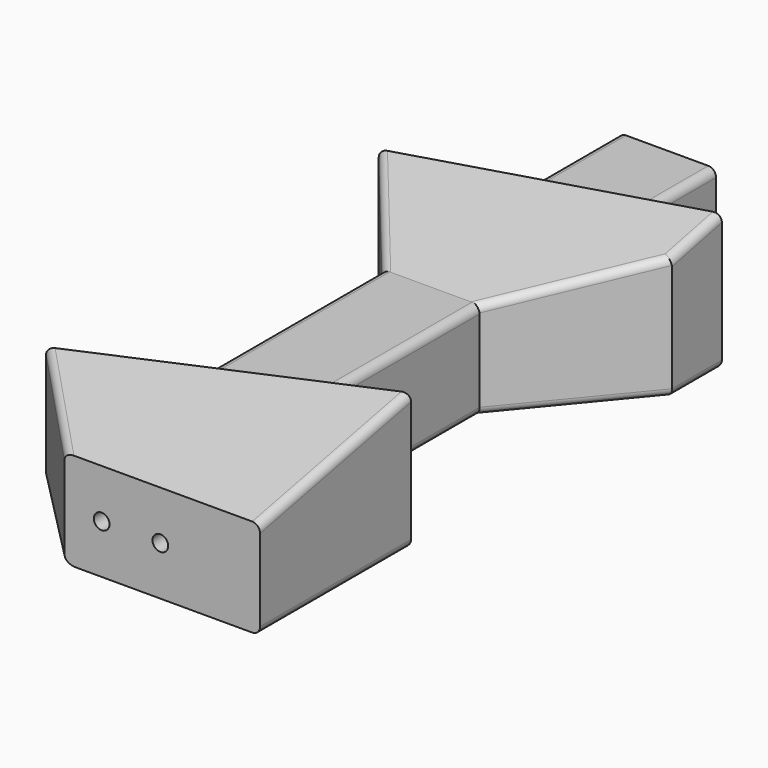
from build123d import *

# Parameters (mm, degrees)
F0_W           = 25
F0_H           = 33
F1_DEPTH       = 25
F3_DEPTH       = 10
F5_DEPTH       = 81.7
F7_DEPTH       = 10
F9_DEPTH       = 92
F10_W          = 13
F10_H          = 13
F11_DEPTH      = 135
F14_W          = 99.2073006928
F14_H          = 199.154949747
F15_DEPTH      = 88
F16_R          = 1.9
F17_DEPTH      = 7
F18_R          = 1.9
F19_DEPTH      = 7
F21_DEPTH      = 18
F22_T1_DEPTH   = 58.2865340729
F22_T3_DEPTH   = 59.3111485648
F22_T5_DEPTH   = 45.6084808239
F22_T7_DEPTH   = 44.6581070284
F22_T9_DEPTH   = 26.3114146799
F22_T11_DEPTH  = 25.9417421253
F22_T16_DEPTH  = 70.8165659944
F22_T23_DEPTH  = 70.8165659944
F22_T29_DEPTH  = 70.8165659944
F22_T35_DEPTH  = 78.4598330308
F22_T41_DEPTH  = 78.4598330308
F22_T47_DEPTH  = 78.4598330308
F22_T54_DEPTH  = 70.8165659944
F22_T60_DEPTH  = 78.4598330308
F22_T66_DEPTH  = 49.2253281189
F22_T71_DEPTH  = 48.4985768834
F22_T77_DEPTH  = 48.4985768834
F22_T83_DEPTH  = 48.4985768834
F22_T89_DEPTH  = 49.2253281189
F22_T94_DEPTH  = 48.4985768834
F22_T100_DEPTH = 48.4985768834
F22_T106_DEPTH = 48.4985768834
F22_T112_DEPTH = 44.6860859582
F22_T117_DEPTH = 50
F22_T122_DEPTH = 44.6860859582
F22_T127_DEPTH = 50
F22_T133_DEPTH = 70.8165659944
F22_T138_DEPTH = 48.4985768834
F22_T146_DEPTH = 48.4985768834
F22_T151_DEPTH = 78.4598330308
F22_T159_DEPTH = 70.8165659944
F22_T163_DEPTH = 49.2253281189
F22_T170_DEPTH = 49.2253281189
F22_T174_DEPTH = 78.4598330308


# Not quite as in the source:
# - a fillet or chamfer that OpenCascade refuses, or shapes differently, is made with other operations: its cross-section is extruded or revolved along the edge and cut away or added


with BuildPart() as f1:
    # F0 (on Top) → F1 (new body)
    with BuildSketch(Plane.XY):
        with Locations((12.5, 16.5)):
            Rectangle(F0_W, F0_H)
        Polygon((-25, 25.3567329635), (0, 0), (0, 33), align=None)
        with Locations((37.5, 16.5)):
            Rectangle(F0_W, F0_H)
        Polygon((25, 40.6432670365), (0, 33), (25, 33), align=None)
        Polygon((0, 101.4598330308), (0, 33), (25, 40.6432670365), (25, 101.4598330308), (25, 137), (0, 137), align=None)
        Polygon((25, 40.6432670365), (25, 33), (50, 33), (50, 48.2865340729), align=None)
        Polygon((-25, 131.6860859582), (0, 101.4598330308), (0, 137), align=None)
        Polygon((25, 137), (25, 101.4598330308), (50, 131.6860859582), (50, 147.6278280835), (25, 142.3139140418), align=None)
        Polygon((25, 142.3139140418), (0, 137), (25, 137), align=None)
        Polygon((0, 177), (0, 137), (25, 142.3139140418), (25, 177), align=None)
    extrude(amount=F1_DEPTH)

    # F2 (on face) → F3 (join)
    with BuildSketch(Plane(origin=(0, 0, 0), x_dir=(1, 0, 0), z_dir=(0, 0, -1))):
        Polygon((50, -131.6860859582), (25, -101.4598330308), (0, -101.4598330308), (-25, -131.6860859582), (50, -147.6278280835), align=None)
    extrude(amount=F3_DEPTH)

    # F4 (on face) → F5 (cut, symmetric)
    with BuildSketch(Plane.YZ.offset(25)):
        Polygon((101.4598330308, -21.1370438337), (147.6278330308, -10), (101.4598330308, 0), align=None)
    extrude(amount=F5_DEPTH, both=True, mode=Mode.SUBTRACT)

    # F6 (on face) → F7 (join)
    with BuildSketch(Plane(origin=(0, 0, 0), x_dir=(1, 0, 0), z_dir=(0, 0, -1))):
        Polygon((50, -48.2865340729), (50, 0), (0, 0), (-25, -25.3567329635), align=None)
    extrude(amount=F7_DEPTH)

    # F8 (on face) → F9 (cut)
    with BuildSketch(Plane.YZ.offset(50)):
        Polygon((48.2865340729, -10), (0, 0), (0, -39.534393698), (48.2865340729, -39.534393698), align=None)
    extrude(amount=-F9_DEPTH, mode=Mode.SUBTRACT)

    # F10 (on face) → F11 (cut)
    with BuildSketch(Plane(origin=(0, 177, 0), x_dir=(-1, 0, 0), z_dir=(0, 1, 0))):
        with Locations((-12.5, 12.5)):
            Rectangle(F10_W, F10_H)
    extrude(amount=-F11_DEPTH, mode=Mode.SUBTRACT)


with BuildPart() as f13_1:
    # F13: instance of F1
    add(f1.part.mirror(Plane(origin=(16.2715907381, 80.4050719696, 50), x_dir=(1, 0, 0), z_dir=(0, 0, 1))))

    # F16 (on face) → F17 (cut)
    with BuildSketch(Plane(origin=(-27.8614600507, 131.0778638485, 0), x_dir=(-0.9781476007, -0.2079116908, 0), z_dir=(-0.2079116908, 0.9781476007, 0))):
        with Locations((-18.6253867704, 87.5)):
            Circle(F16_R)
        with BuildLine():
            ThreePointArc((-72.2009313853, 87.5), (-70.3009313853, 85.6), (-68.4009313853, 87.5))
            ThreePointArc((-68.4009313853, 87.5), (-70.3009313853, 89.4), (-72.2009313853, 87.5))
        make_face()
    extrude(amount=-F17_DEPTH, mode=Mode.SUBTRACT)

    # F18 (on face) → F19 (cut)
    with BuildSketch(Plane(origin=(-9.2266829073, 30.1791199472, 0), x_dir=(-0.956304756, -0.2923717047, 0), z_dir=(-0.2923717047, 0.956304756, 0))):
        with Locations((0.6940276563, 87.5)):
            Circle(F18_R)
        with BuildLine():
            ThreePointArc((-54.6328540802, 87.5), (-52.7328540802, 85.6), (-50.8328540802, 87.5))
            ThreePointArc((-50.8328540802, 87.5), (-52.7328540802, 89.4), (-54.6328540802, 87.5))
        make_face()
    extrude(amount=-F19_DEPTH, mode=Mode.SUBTRACT)

    # F20 (on face) → F21 (cut)
    with BuildSketch(Plane.XZ):
        with BuildLine():
            ThreePointArc((11.5, 87.5), (9.5, 89.5), (7.5, 87.5))
            Line((7.5, 87.5), (9.5, 87.5))
            Line((9.5, 87.5), (11.5, 87.5))
        make_face()
        with BuildLine():
            ThreePointArc((26.5, 87.5), (24.5, 89.5), (22.5, 87.5))
            ThreePointArc((22.5, 87.5), (24.5, 85.5), (26.5, 87.5))
        make_face()
        with BuildLine():
            Line((9.5, 87.5), (7.5, 87.5))
            ThreePointArc((7.5, 87.5), (9.5, 85.5), (11.5, 87.5))
            Line((11.5, 87.5), (9.5, 87.5))
        make_face()
    extrude(amount=-F21_DEPTH, mode=Mode.SUBTRACT)

    # F22: fillet of radius 2 on 18 edges, made by hand

    # F22_s2 → F22_t1 (cut)
    with BuildSketch(Plane.XZ.offset(-53.2865340729)):
        with BuildLine():
            ThreePointArc((48, 75), (49.4142135624, 75.5857864376), (50, 77))
            Line((50, 77), (50, 75))
            Line((50, 75), (48, 75))
        make_face()
    extrude(amount=F22_T1_DEPTH, mode=Mode.SUBTRACT)

    # F22_s4 → F22_t3 (cut)
    with BuildSketch(Plane(origin=(0, 73.0406545768, 15.1265059668), x_dir=(1, 0, 0), z_dir=(0, -0.9792214434, -0.2027938973))):
        with BuildLine():
            ThreePointArc((48, 97.9221443392), (49.4142135624, 97.3363579016), (50, 95.9221443392))
            Line((50, 95.9221443392), (50, 97.9221443392))
            Line((50, 97.9221443392), (48, 97.9221443392))
        make_face()
    extrude(amount=F22_T3_DEPTH, mode=Mode.SUBTRACT)

    # F22_s6 → F22_t5 (cut)
    with BuildSketch(Plane(origin=(-28.5103996887, 28.9172236636, 0), x_dir=(0, 0, 1), z_dir=(0.7020799377, -0.71209814, 0))):
        with BuildLine():
            ThreePointArc((77, 0), (75.5857864376, -0.5857864376), (75, -2))
            Line((75, -2), (75, 0))
            Line((75, 0), (77, 0))
        make_face()
    extrude(amount=F22_T5_DEPTH, mode=Mode.SUBTRACT)

    # F22_s8 → F22_t7 (cut)
    with BuildSketch(Plane(origin=(-38.1424676079, 38.6867346281, 8.0119096081), x_dir=(0.71209814, 0.7020799377, 0), z_dir=(0.6945676893, -0.7044786969, -0.145895478))):
        with BuildLine():
            ThreePointArc((0, 97.1971020036), (0.4884593774, 98.5067756066), (1.7152449464, 99.1767268568))
            Line((1.7152449464, 99.1767268568), (0, 98.9300009856))
            Line((0, 98.9300009856), (0, 97.1971020036))
        make_face()
    extrude(amount=F22_T7_DEPTH, mode=Mode.SUBTRACT)

    # F22_s10 → F22_t9 (cut)
    with BuildSketch(Plane(origin=(0, 142.94202974, 30.9612783183), x_dir=(1, 0, 0), z_dir=(0, 0.9773365731, 0.2116913388))):
        with BuildLine():
            ThreePointArc((50, -74.2554894164), (49.4142135624, -75.6697029788), (48, -76.2554894164))
            Line((48, -76.2554894164), (50, -76.2554894164))
            Line((50, -76.2554894164), (50, -74.2554894164))
        make_face()
    extrude(amount=F22_T9_DEPTH, mode=Mode.SUBTRACT)

    # F22_s12 → F22_t11 (cut)
    with BuildSketch(Plane.XZ.offset(-152.6278280835)):
        with BuildLine():
            ThreePointArc((48, 75), (49.4142135624, 75.5857864376), (50, 77))
            Line((50, 77), (50, 75))
            Line((50, 75), (48, 75))
        make_face()
    extrude(amount=F22_T11_DEPTH, mode=Mode.SUBTRACT)


with BuildPart() as f1_1:
    add(f1.part)

    # F14 (on offset) → F15 (cut)
    with BuildSketch(Plane.XY.offset(50)):
        with Locations((12.7710904926, 90.3895613737)):
            Rectangle(F14_W, F14_H)
    extrude(amount=-F15_DEPTH, mode=Mode.SUBTRACT)


with BuildPart() as f22_tool14:
    # F22_s15 → F22_t16 (new body)
    with BuildSketch(Plane.XZ.offset(-35.6432670365)):
        with BuildLine():
            ThreePointArc((25, 98), (24.4142135624, 99.4142135624), (23, 100))
            Line((23, 100), (25, 100))
            Line((25, 100), (25, 98))
        make_face()
    extrude(amount=-F22_T16_DEPTH)

    split(bisect_by=Plane(origin=(-9.2266829073, 30.1791199472, 0), x_dir=(0, 0, 1), z_dir=(-0.2923717047, 0.956304756, 0)), keep=Keep.TOP)

    split(bisect_by=Plane(origin=(-34.9845202296, 28.9355418232, 0), x_dir=(0, 0, 1), z_dir=(0.7705799894, -0.6373432983, 0)), keep=Keep.TOP)

    split(bisect_by=Plane(origin=(0, -16.1426266471, 74.5272787043), x_dir=(1, 0, 0), z_dir=(0, -0.2116913388, 0.9773365731)), keep=Keep.TOP)


with BuildPart() as f13_1_1:
    add(f13_1.part)

    # F22_t13: cut F22_tool14
    add(f22_tool14.part, mode=Mode.SUBTRACT)


with BuildPart() as f22_tool21:
    # F22_s22 → F22_t23 (new body)
    with BuildSketch(Plane.XZ.offset(-35.6432670365)):
        with BuildLine():
            ThreePointArc((25, 98), (24.4142135624, 99.4142135624), (23, 100))
            Line((23, 100), (25, 100))
            Line((25, 100), (25, 98))
        make_face()
    extrude(amount=-F22_T23_DEPTH)

    split(bisect_by=Plane(origin=(-34.9845202296, 28.9355418232, 0), x_dir=(0, 0, 1), z_dir=(-0.7705799894, 0.6373432983, 0)), keep=Keep.TOP)

    split(bisect_by=Plane(origin=(0, -16.1426266471, 74.5272787043), x_dir=(1, 0, 0), z_dir=(0, -0.2116913388, 0.9773365731)), keep=Keep.TOP)


with BuildPart() as f13_1_2:
    add(f13_1_1.part)

    # F22_t20: cut F22_tool21
    add(f22_tool21.part, mode=Mode.SUBTRACT)


with BuildPart() as f22_tool27:
    # F22_s28 → F22_t29 (new body)
    with BuildSketch(Plane.XZ.offset(-35.6432670365)):
        with BuildLine():
            ThreePointArc((25, 98), (24.4142135624, 99.4142135624), (23, 100))
            Line((23, 100), (25, 100))
            Line((25, 100), (25, 98))
        make_face()
    extrude(amount=-F22_T29_DEPTH)

    split(bisect_by=Plane(origin=(-34.9845202296, 28.9355418232, 0), x_dir=(0, 0, 1), z_dir=(0.7705799894, -0.6373432983, 0)), keep=Keep.TOP)

    split(bisect_by=Plane(origin=(0, -16.1426266471, 74.5272787043), x_dir=(1, 0, 0), z_dir=(0, 0.2116913388, -0.9773365731)), keep=Keep.TOP)


with BuildPart() as f13_1_3:
    add(f13_1_2.part)

    # F22_t26: cut F22_tool27
    add(f22_tool27.part, mode=Mode.SUBTRACT)


with BuildPart() as f22_tool33:
    # F22_s34 → F22_t35 (new body)
    with BuildSketch(Plane.XZ.offset(-106.4598330308)):
        with BuildLine():
            ThreePointArc((0, 98), (0.5857864376, 99.4142135624), (2, 100))
            Line((2, 100), (0, 100))
            Line((0, 100), (0, 98))
        make_face()
    extrude(amount=F22_T35_DEPTH)

    split(bisect_by=Plane(origin=(49.8293582326, 41.2136416249, 0), x_dir=(0, 0, 1), z_dir=(0.7705799894, 0.6373432983, 0)), keep=Keep.TOP)

    split(bisect_by=Plane(origin=(0, -16.1426266471, 74.5272787043), x_dir=(1, 0, 0), z_dir=(0, -0.2116913388, 0.9773365731)), keep=Keep.TOP)


with BuildPart() as f13_1_4:
    add(f13_1_3.part)

    # F22_t32: cut F22_tool33
    add(f22_tool33.part, mode=Mode.SUBTRACT)


with BuildPart() as f22_tool39:
    # F22_s40 → F22_t41 (new body)
    with BuildSketch(Plane.XZ.offset(-106.4598330308)):
        with BuildLine():
            ThreePointArc((0, 98), (0.5857864376, 99.4142135624), (2, 100))
            Line((2, 100), (0, 100))
            Line((0, 100), (0, 98))
        make_face()
    extrude(amount=F22_T41_DEPTH)

    split(bisect_by=Plane(origin=(49.8293582326, 41.2136416249, 0), x_dir=(0, 0, 1), z_dir=(-0.7705799894, -0.6373432983, 0)), keep=Keep.TOP)

    split(bisect_by=Plane(origin=(0, -16.1426266471, 74.5272787043), x_dir=(1, 0, 0), z_dir=(0, 0.2116913388, -0.9773365731)), keep=Keep.TOP)


with BuildPart() as f13_1_5:
    add(f13_1_4.part)

    # F22_t38: cut F22_tool39
    add(f22_tool39.part, mode=Mode.SUBTRACT)


with BuildPart() as f22_tool45:
    # F22_s46 → F22_t47 (new body)
    with BuildSketch(Plane.XZ.offset(-106.4598330308)):
        with BuildLine():
            ThreePointArc((0, 98), (0.5857864376, 99.4142135624), (2, 100))
            Line((2, 100), (0, 100))
            Line((0, 100), (0, 98))
        make_face()
    extrude(amount=F22_T47_DEPTH)

    split(bisect_by=Plane(origin=(-9.2266829073, 30.1791199472, 0), x_dir=(0, 0, 1), z_dir=(-0.2923717047, 0.956304756, 0)), keep=Keep.TOP)

    split(bisect_by=Plane(origin=(49.8293582326, 41.2136416249, 0), x_dir=(0, 0, 1), z_dir=(-0.7705799894, -0.6373432983, 0)), keep=Keep.TOP)

    split(bisect_by=Plane(origin=(0, -16.1426266471, 74.5272787043), x_dir=(1, 0, 0), z_dir=(0, -0.2116913388, 0.9773365731)), keep=Keep.TOP)


with BuildPart() as f13_1_6:
    add(f13_1_5.part)

    # F22_t44: cut F22_tool45
    add(f22_tool45.part, mode=Mode.SUBTRACT)


with BuildPart() as f22_tool52:
    # F22_s53 → F22_t54 (new body)
    with BuildSketch(Plane.XZ.offset(-35.6432670365)):
        with BuildLine():
            ThreePointArc((23, 75), (24.4142135624, 75.5857864376), (25, 77))
            Line((25, 77), (25, 75))
            Line((25, 75), (23, 75))
        make_face()
    extrude(amount=-F22_T54_DEPTH)

    split(bisect_by=Plane(origin=(-9.2266829073, 30.1791199472, 0), x_dir=(0, 0, 1), z_dir=(-0.2923717047, 0.956304756, 0)), keep=Keep.TOP)

    split(bisect_by=Plane(origin=(-34.9845202296, 28.9355418232, 0), x_dir=(0, 0, 1), z_dir=(0.7705799894, -0.6373432983, 0)), keep=Keep.TOP)


with BuildPart() as f13_1_7:
    add(f13_1_6.part)

    # F22_t51: cut F22_tool52
    add(f22_tool52.part, mode=Mode.SUBTRACT)


with BuildPart() as f22_tool58:
    # F22_s59 → F22_t60 (new body)
    with BuildSketch(Plane.XZ.offset(-106.4598330308)):
        with BuildLine():
            ThreePointArc((2, 75), (0.5857864376, 75.5857864376), (0, 77))
            Line((0, 77), (0, 75))
            Line((0, 75), (2, 75))
        make_face()
    extrude(amount=F22_T60_DEPTH)

    split(bisect_by=Plane(origin=(-9.2266829073, 30.1791199472, 0), x_dir=(0, 0, 1), z_dir=(-0.2923717047, 0.956304756, 0)), keep=Keep.TOP)

    split(bisect_by=Plane(origin=(49.8293582326, 41.2136416249, 0), x_dir=(0, 0, 1), z_dir=(-0.7705799894, -0.6373432983, 0)), keep=Keep.TOP)


with BuildPart() as f13_1_8:
    add(f13_1_7.part)

    # F22_t57: cut F22_tool58
    add(f22_tool58.part, mode=Mode.SUBTRACT)


with BuildPart() as f22_tool64:
    # F22_s65 → F22_t66 (new body)
    with BuildSketch(Plane(origin=(-78.016074724, 94.3253442805, 0), x_dir=(0, 0, 1), z_dir=(0.6373432983, -0.7705799894, 0))):
        with BuildLine():
            ThreePointArc((75, -66.6647446284), (75.5857864376, -65.250531066), (77, -64.6647446284))
            Line((77, -64.6647446284), (75, -64.6647446284))
            Line((75, -64.6647446284), (75, -66.6647446284))
        make_face()
    extrude(amount=F22_T66_DEPTH)

    split(bisect_by=Plane.YZ, keep=Keep.BOTTOM)


with BuildPart() as f13_1_9:
    add(f13_1_8.part)

    # F22_t63: cut F22_tool64
    add(f22_tool64.part, mode=Mode.SUBTRACT)


with BuildPart() as f22_tool69:
    # F22_s70 → F22_t71 (new body)
    with BuildSketch(Plane(origin=(-86.5725065584, 104.6704991917, 22.6716555172), x_dir=(0.7705799894, 0.6373432983, 0), z_dir=(0.6286469564, -0.7600656763, -0.1646304099))):
        with BuildLine():
            ThreePointArc((64.6647446284, 84.0181212592), (65.1581457726, 85.3334766818), (66.3949045162, 85.9998342338))
            Line((66.3949045162, 85.9998342338), (64.6647446284, 85.7642468686))
            Line((64.6647446284, 85.7642468686), (64.6647446284, 84.0181212592))
        make_face()
    extrude(amount=F22_T71_DEPTH)

    split(bisect_by=Plane.YZ, keep=Keep.BOTTOM)

    split(bisect_by=Plane.XY.offset(100), keep=Keep.TOP)


with BuildPart() as f13_1_10:
    add(f13_1_9.part)

    # F22_t68: cut F22_tool69
    add(f22_tool69.part, mode=Mode.SUBTRACT)


with BuildPart() as f22_tool75:
    # F22_s76 → F22_t77 (new body)
    with BuildSketch(Plane(origin=(-86.5725065584, 104.6704991917, 22.6716555172), x_dir=(0.7705799894, 0.6373432983, 0), z_dir=(0.6286469564, -0.7600656763, -0.1646304099))):
        with BuildLine():
            ThreePointArc((64.6647446284, 84.0181212592), (65.1581457726, 85.3334766818), (66.3949045162, 85.9998342338))
            Line((66.3949045162, 85.9998342338), (64.6647446284, 85.7642468686))
            Line((64.6647446284, 85.7642468686), (64.6647446284, 84.0181212592))
        make_face()
    extrude(amount=F22_T77_DEPTH)

    split(bisect_by=Plane.YZ, keep=Keep.TOP)

    split(bisect_by=Plane.XY.offset(100), keep=Keep.TOP)


with BuildPart() as f13_1_11:
    add(f13_1_10.part)

    # F22_t74: cut F22_tool75
    add(f22_tool75.part, mode=Mode.SUBTRACT)


with BuildPart() as f22_tool81:
    # F22_s82 → F22_t83 (new body)
    with BuildSketch(Plane(origin=(-86.5725065584, 104.6704991917, 22.6716555172), x_dir=(0.7705799894, 0.6373432983, 0), z_dir=(0.6286469564, -0.7600656763, -0.1646304099))):
        with BuildLine():
            ThreePointArc((64.6647446284, 84.0181212592), (65.1581457726, 85.3334766818), (66.3949045162, 85.9998342338))
            Line((66.3949045162, 85.9998342338), (64.6647446284, 85.7642468686))
            Line((64.6647446284, 85.7642468686), (64.6647446284, 84.0181212592))
        make_face()
    extrude(amount=F22_T83_DEPTH)

    split(bisect_by=Plane.YZ, keep=Keep.BOTTOM)

    split(bisect_by=Plane.XY.offset(100), keep=Keep.BOTTOM)


with BuildPart() as f13_1_12:
    add(f13_1_11.part)

    # F22_t80: cut F22_tool81
    add(f22_tool81.part, mode=Mode.SUBTRACT)


with BuildPart() as f22_tool87:
    # F22_s88 → F22_t89 (new body)
    with BuildSketch(Plane(origin=(56.7978037382, 68.6713912604, 0), x_dir=(0, 0, 1), z_dir=(0.6373432983, 0.7705799894, 0))):
        with BuildLine():
            ThreePointArc((75, -47.4002448925), (75.5857864376, -45.9860313302), (77, -45.4002448925))
            Line((77, -45.4002448925), (75, -45.4002448925))
            Line((75, -45.4002448925), (75, -47.4002448925))
        make_face()
    extrude(amount=F22_T89_DEPTH)

    split(bisect_by=Plane.YZ.offset(25), keep=Keep.TOP)


with BuildPart() as f13_1_13:
    add(f13_1_12.part)

    # F22_t86: cut F22_tool87
    add(f22_tool87.part, mode=Mode.SUBTRACT)


with BuildPart() as f22_tool92:
    # F22_s93 → F22_t94 (new body)
    with BuildSketch(Plane(origin=(65.9639487049, 79.7537199058, 17.2746750792), x_dir=(-0.7705799894, 0.6373432983, 0), z_dir=(0.6286469564, 0.7600656763, 0.1646304099))):
        with BuildLine():
            ThreePointArc((45.4002448925, 81.3949690485), (45.8936460368, 82.7103244711), (47.1304047803, 83.3766820231))
            Line((47.1304047803, 83.3766820231), (45.4002448925, 83.1410946579))
            Line((45.4002448925, 83.1410946579), (45.4002448925, 81.3949690485))
        make_face()
    extrude(amount=F22_T94_DEPTH)

    split(bisect_by=Plane.YZ.offset(25), keep=Keep.BOTTOM)

    split(bisect_by=Plane.XY.offset(100), keep=Keep.TOP)


with BuildPart() as f13_1_14:
    add(f13_1_13.part)

    # F22_t91: cut F22_tool92
    add(f22_tool92.part, mode=Mode.SUBTRACT)


with BuildPart() as f22_tool98:
    # F22_s99 → F22_t100 (new body)
    with BuildSketch(Plane(origin=(65.9639487049, 79.7537199058, 17.2746750792), x_dir=(-0.7705799894, 0.6373432983, 0), z_dir=(0.6286469564, 0.7600656763, 0.1646304099))):
        with BuildLine():
            ThreePointArc((45.4002448925, 81.3949690485), (45.8936460368, 82.7103244711), (47.1304047803, 83.3766820231))
            Line((47.1304047803, 83.3766820231), (45.4002448925, 83.1410946579))
            Line((45.4002448925, 83.1410946579), (45.4002448925, 81.3949690485))
        make_face()
    extrude(amount=F22_T100_DEPTH)

    split(bisect_by=Plane.YZ.offset(25), keep=Keep.TOP)

    split(bisect_by=Plane.XY.offset(100), keep=Keep.BOTTOM)


with BuildPart() as f13_1_15:
    add(f13_1_14.part)

    # F22_t97: cut F22_tool98
    add(f22_tool98.part, mode=Mode.SUBTRACT)


with BuildPart() as f22_tool104:
    # F22_s105 → F22_t106 (new body)
    with BuildSketch(Plane(origin=(65.9639487049, 79.7537199058, 17.2746750792), x_dir=(-0.7705799894, 0.6373432983, 0), z_dir=(0.6286469564, 0.7600656763, 0.1646304099))):
        with BuildLine():
            ThreePointArc((45.4002448925, 81.3949690485), (45.8936460368, 82.7103244711), (47.1304047803, 83.3766820231))
            Line((47.1304047803, 83.3766820231), (45.4002448925, 83.1410946579))
            Line((45.4002448925, 83.1410946579), (45.4002448925, 81.3949690485))
        make_face()
    extrude(amount=F22_T106_DEPTH)

    split(bisect_by=Plane.YZ.offset(25), keep=Keep.TOP)

    split(bisect_by=Plane.XY.offset(100), keep=Keep.TOP)


with BuildPart() as f13_1_16:
    add(f13_1_15.part)

    # F22_t103: cut F22_tool104
    add(f22_tool104.part, mode=Mode.SUBTRACT)


with BuildPart() as f22_tool110:
    # F22_s111 → F22_t112 (new body)
    with BuildSketch(Plane.XZ.offset(-137.3139140418)):
        with BuildLine():
            ThreePointArc((25, 98), (24.4142135624, 99.4142135624), (23, 100))
            Line((23, 100), (25, 100))
            Line((25, 100), (25, 98))
        make_face()
    extrude(amount=-F22_T112_DEPTH)

    split(bisect_by=Plane(origin=(-27.8614600507, 131.0778638485, 0), x_dir=(0, 0, 1), z_dir=(-0.2079116908, 0.9781476007, 0)), keep=Keep.TOP)


with BuildPart() as f13_1_17:
    add(f13_1_16.part)

    # F22_t109: cut F22_tool110
    add(f22_tool110.part, mode=Mode.SUBTRACT)


with BuildPart() as f22_tool115:
    # F22_s116 → F22_t117 (new body)
    with BuildSketch(Plane.XZ.offset(-182)):
        with BuildLine():
            ThreePointArc((2, 75), (0.5857864376, 75.5857864376), (0, 77))
            Line((0, 77), (0, 75))
            Line((0, 75), (2, 75))
        make_face()
    extrude(amount=F22_T117_DEPTH)

    split(bisect_by=Plane(origin=(-27.8614600507, 131.0778638485, 0), x_dir=(0, 0, 1), z_dir=(-0.2079116908, 0.9781476007, 0)), keep=Keep.TOP)


with BuildPart() as f13_1_18:
    add(f13_1_17.part)

    # F22_t114: cut F22_tool115
    add(f22_tool115.part, mode=Mode.SUBTRACT)


with BuildPart() as f22_tool120:
    # F22_s121 → F22_t122 (new body)
    with BuildSketch(Plane.XZ.offset(-137.3139140418)):
        with BuildLine():
            ThreePointArc((23, 75), (24.4142135624, 75.5857864376), (25, 77))
            Line((25, 77), (25, 75))
            Line((25, 75), (23, 75))
        make_face()
    extrude(amount=-F22_T122_DEPTH)

    split(bisect_by=Plane(origin=(-27.8614600507, 131.0778638485, 0), x_dir=(0, 0, 1), z_dir=(-0.2079116908, 0.9781476007, 0)), keep=Keep.TOP)


with BuildPart() as f13_1_19:
    add(f13_1_18.part)

    # F22_t119: cut F22_tool120
    add(f22_tool120.part, mode=Mode.SUBTRACT)


with BuildPart() as f22_tool125:
    # F22_s126 → F22_t127 (new body)
    with BuildSketch(Plane.XZ.offset(-182)):
        with BuildLine():
            ThreePointArc((0, 98), (0.5857864376, 99.4142135624), (2, 100))
            Line((2, 100), (0, 100))
            Line((0, 100), (0, 98))
        make_face()
    extrude(amount=F22_T127_DEPTH)

    split(bisect_by=Plane(origin=(-27.8614600507, 131.0778638485, 0), x_dir=(0, 0, 1), z_dir=(-0.2079116908, 0.9781476007, 0)), keep=Keep.TOP)


with BuildPart() as f13_1_20:
    add(f13_1_19.part)

    # F22_t124: cut F22_tool125
    add(f22_tool125.part, mode=Mode.SUBTRACT)


with BuildPart() as f22_tool131:
    # F22_s132 → F22_t133 (new body)
    with BuildSketch(Plane.XZ.offset(-35.6432670365)):
        with BuildLine():
            ThreePointArc((25, 98), (24.4142135624, 99.4142135624), (23, 100))
            Line((23, 100), (25, 100))
            Line((25, 100), (25, 98))
        make_face()
    extrude(amount=-F22_T133_DEPTH)

    split(bisect_by=Plane(origin=(-34.9845202296, 28.9355418232, 0), x_dir=(0, 0, 1), z_dir=(-0.7705799894, 0.6373432983, 0)), keep=Keep.TOP)

    split(bisect_by=Plane(origin=(0, -16.1426266471, 74.5272787043), x_dir=(1, 0, 0), z_dir=(0, 0.2116913388, -0.9773365731)), keep=Keep.TOP)


with BuildPart() as f22_tool136:
    # F22_s137 → F22_t138 (new body)
    with BuildSketch(Plane(origin=(65.9639487049, 79.7537199058, 17.2746750792), x_dir=(-0.7705799894, 0.6373432983, 0), z_dir=(0.6286469564, 0.7600656763, 0.1646304099))):
        with BuildLine():
            ThreePointArc((45.4002448925, 81.3949690485), (45.8936460368, 82.7103244711), (47.1304047803, 83.3766820231))
            Line((47.1304047803, 83.3766820231), (45.4002448925, 83.1410946579))
            Line((45.4002448925, 83.1410946579), (45.4002448925, 81.3949690485))
        make_face()
    extrude(amount=F22_T138_DEPTH)

    split(bisect_by=Plane.YZ.offset(25), keep=Keep.BOTTOM)

    split(bisect_by=Plane.XY.offset(100), keep=Keep.BOTTOM)


with BuildPart() as f22_tool131_1:
    add(f22_tool131.part)

    # F22_t141: intersect F22_tool136
    add(f22_tool136.part, mode=Mode.INTERSECT)


with BuildPart() as f13_1_21:
    add(f13_1_20.part)

    # F22_t129: cut F22_tool131
    add(f22_tool131_1.part, mode=Mode.SUBTRACT)


with BuildPart() as f22_tool144:
    # F22_s145 → F22_t146 (new body)
    with BuildSketch(Plane(origin=(-86.5725065584, 104.6704991917, 22.6716555172), x_dir=(0.7705799894, 0.6373432983, 0), z_dir=(0.6286469564, -0.7600656763, -0.1646304099))):
        with BuildLine():
            ThreePointArc((64.6647446284, 84.0181212592), (65.1581457726, 85.3334766818), (66.3949045162, 85.9998342338))
            Line((66.3949045162, 85.9998342338), (64.6647446284, 85.7642468686))
            Line((64.6647446284, 85.7642468686), (64.6647446284, 84.0181212592))
        make_face()
    extrude(amount=F22_T146_DEPTH)

    split(bisect_by=Plane.YZ, keep=Keep.TOP)

    split(bisect_by=Plane.XY.offset(100), keep=Keep.BOTTOM)


with BuildPart() as f22_tool149:
    # F22_s150 → F22_t151 (new body)
    with BuildSketch(Plane.XZ.offset(-106.4598330308)):
        with BuildLine():
            ThreePointArc((0, 98), (0.5857864376, 99.4142135624), (2, 100))
            Line((2, 100), (0, 100))
            Line((0, 100), (0, 98))
        make_face()
    extrude(amount=F22_T151_DEPTH)

    split(bisect_by=Plane(origin=(49.8293582326, 41.2136416249, 0), x_dir=(0, 0, 1), z_dir=(0.7705799894, 0.6373432983, 0)), keep=Keep.TOP)

    split(bisect_by=Plane(origin=(0, -16.1426266471, 74.5272787043), x_dir=(1, 0, 0), z_dir=(0, 0.2116913388, -0.9773365731)), keep=Keep.TOP)


with BuildPart() as f22_tool144_1:
    add(f22_tool144.part)

    # F22_t154: intersect F22_tool149
    add(f22_tool149.part, mode=Mode.INTERSECT)


with BuildPart() as f13_1_22:
    add(f13_1_21.part)

    # F22_t142: cut F22_tool144
    add(f22_tool144_1.part, mode=Mode.SUBTRACT)


with BuildPart() as f22_tool157:
    # F22_s158 → F22_t159 (new body)
    with BuildSketch(Plane.XZ.offset(-35.6432670365)):
        with BuildLine():
            ThreePointArc((23, 75), (24.4142135624, 75.5857864376), (25, 77))
            Line((25, 77), (25, 75))
            Line((25, 75), (23, 75))
        make_face()
    extrude(amount=-F22_T159_DEPTH)

    split(bisect_by=Plane(origin=(-34.9845202296, 28.9355418232, 0), x_dir=(0, 0, 1), z_dir=(-0.7705799894, 0.6373432983, 0)), keep=Keep.TOP)


with BuildPart() as f22_tool161:
    # F22_s162 → F22_t163 (new body)
    with BuildSketch(Plane(origin=(56.7978037382, 68.6713912604, 0), x_dir=(0, 0, 1), z_dir=(0.6373432983, 0.7705799894, 0))):
        with BuildLine():
            ThreePointArc((75, -47.4002448925), (75.5857864376, -45.9860313302), (77, -45.4002448925))
            Line((77, -45.4002448925), (75, -45.4002448925))
            Line((75, -45.4002448925), (75, -47.4002448925))
        make_face()
    extrude(amount=F22_T163_DEPTH)

    split(bisect_by=Plane.YZ.offset(25), keep=Keep.BOTTOM)


with BuildPart() as f22_tool157_1:
    add(f22_tool157.part)

    # F22_t165: intersect F22_tool161
    add(f22_tool161.part, mode=Mode.INTERSECT)


with BuildPart() as f13_1_23:
    add(f13_1_22.part)

    # F22_t155: cut F22_tool157
    add(f22_tool157_1.part, mode=Mode.SUBTRACT)


with BuildPart() as f22_tool168:
    # F22_s169 → F22_t170 (new body)
    with BuildSketch(Plane(origin=(-78.016074724, 94.3253442805, 0), x_dir=(0, 0, 1), z_dir=(0.6373432983, -0.7705799894, 0))):
        with BuildLine():
            ThreePointArc((75, -66.6647446284), (75.5857864376, -65.250531066), (77, -64.6647446284))
            Line((77, -64.6647446284), (75, -64.6647446284))
            Line((75, -64.6647446284), (75, -66.6647446284))
        make_face()
    extrude(amount=F22_T170_DEPTH)

    split(bisect_by=Plane.YZ, keep=Keep.TOP)


with BuildPart() as f22_tool172:
    # F22_s173 → F22_t174 (new body)
    with BuildSketch(Plane.XZ.offset(-106.4598330308)):
        with BuildLine():
            ThreePointArc((2, 75), (0.5857864376, 75.5857864376), (0, 77))
            Line((0, 77), (0, 75))
            Line((0, 75), (2, 75))
        make_face()
    extrude(amount=F22_T174_DEPTH)

    split(bisect_by=Plane(origin=(49.8293582326, 41.2136416249, 0), x_dir=(0, 0, 1), z_dir=(0.7705799894, 0.6373432983, 0)), keep=Keep.TOP)


with BuildPart() as f22_tool168_1:
    add(f22_tool168.part)

    # F22_t176: intersect F22_tool172
    add(f22_tool172.part, mode=Mode.INTERSECT)


with BuildPart() as f13_1_24:
    add(f13_1_23.part)

    # F22_t166: cut F22_tool168
    add(f22_tool168_1.part, mode=Mode.SUBTRACT)


solid = f13_1_24.part
